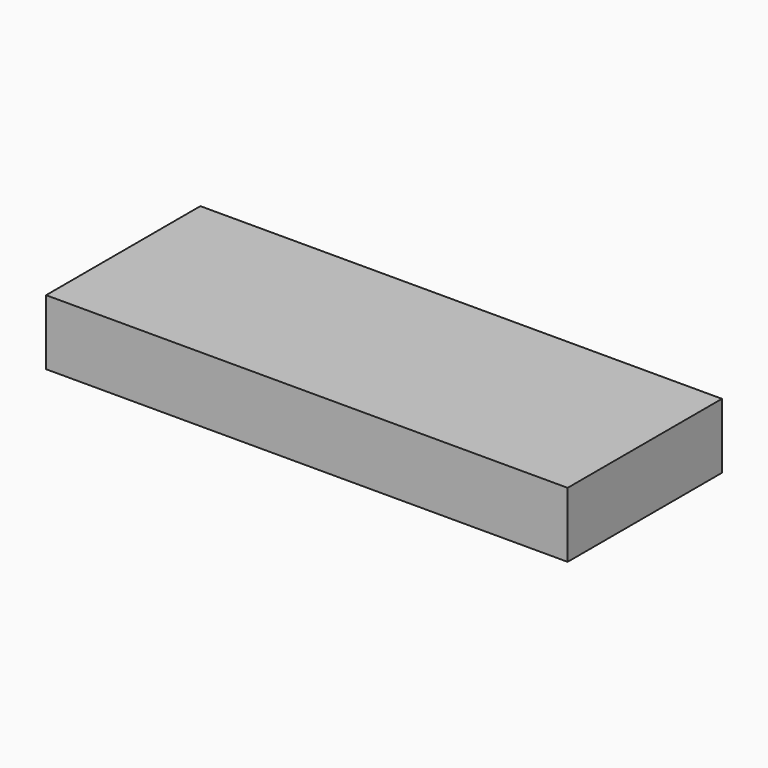
from build123d import *

# Parameters (mm, degrees)
F0_W      = 122.5
F0_H      = 57
F1_DEPTH  = 7
F2_R      = 5
F4_W      = 7.9906114999
F4_H      = 3.491573553
F6_DEPTH  = 0.75
F3_R      = 2.8696252626
F3_R_2    = 3.0222724843
F3_W      = 6.7058205605
F3_H      = 3.0176183209
F7_DEPTH  = 0.75
F5_R      = 4.4116461286
F8_DEPTH  = 0.5
F10_W     = 10.931
F10_H     = 2.55831494
F11_DEPTH = 1
F12_R     = 2.4748812048
F13_DEPTH = 7
F14_W     = 9.2436559498
F14_H     = 3.1246161088
F15_DEPTH = 25


# Not quite as in the source:
# - a fillet or chamfer that OpenCascade refuses, or shapes differently, is made with other operations: its cross-section is extruded or revolved along the edge and cut away or added


with BuildPart() as f1:
    # F0 (on Top) → F1 (new body)
    with BuildSketch(Plane.XY):
        Rectangle(F0_W, F0_H)
    extrude(amount=F1_DEPTH)

    # F2
    f2_edges = [f1.edges().sort_by_distance(p)[0] for p in [
        (61.25, -28.5, 3.5),
        (61.25, 28.5, 3.5),
        (-61.25, -28.5, 3.5),
        (-61.25, 28.5, 3.5),
    ]]
    fillet(f2_edges, radius=F2_R)

    # F4 (on face) → F6 (join)
    with BuildSketch(Plane(origin=(-61.25, 0, 0), x_dir=(0, -1, 0), z_dir=(-1, 0, 0))):
        with Locations((-17.3388376055, 3.4486234912)):
            Rectangle(F4_W, F4_H)
    extrude(amount=F6_DEPTH)

    # F3 (on face) → F7 (join)
    with BuildSketch(Plane.XZ.offset(28.5)):
        with Locations((-42.9149009287, 3.2392428257)):
            Circle(F3_R)
        with Locations((-34.8679199815, 3.2392428257)):
            Circle(F3_R_2)
        with Locations((-51.1295311153, 3.2392428257)):
            Rectangle(F3_W, F3_H)
    extrude(amount=F7_DEPTH)

    # F5 (on face) → F8 (cut)
    with BuildSketch(Plane.XY.offset(7)):
        with Locations((54.2597770691, -0.2932948992)):
            Circle(F5_R)
    extrude(amount=-F8_DEPTH, mode=Mode.SUBTRACT)

    # F9: fillet of radius 1 on 1 edges, made by hand


with BuildPart() as f9_tool2:
    # F9_s3 → F9_t4 (revolve)
    with BuildSketch(Plane.XZ.offset(0.2932948992)):
        with BuildLine():
            ThreePointArc((58.6714231977, 7.5), (58.3785299789, 6.7928932188), (57.6714231977, 6.5))
            Line((57.6714231977, 6.5), (58.6714231977, 6.5))
            Line((58.6714231977, 6.5), (58.6714231977, 7.5))
        make_face()
    revolve(axis=Axis((54.2597770691, -0.2932948992, 6.5), (0, 0, 1)))

    split(bisect_by=Plane.XY.offset(7), keep=Keep.BOTTOM)


with BuildPart() as f1_1:
    add(f1.part)

    # F9_t1: union F9_tool2
    add(f9_tool2.part)

    # F10 (on face) → F11 (join)
    with BuildSketch(Plane.YZ.offset(61.25)):
        with Locations((-0.3508040114, 3.4726482118)):
            Rectangle(F10_W, F10_H)
    extrude(amount=-F11_DEPTH)

    # F12 (on face) → F13 (cut)
    with BuildSketch(Plane.YZ.offset(61.25)):
        with Locations((16.8605856597, 3.6920385901)):
            Circle(F12_R)
    extrude(amount=-F13_DEPTH, mode=Mode.SUBTRACT)

    # F14 (on face) → F15 (intersect)
    with BuildSketch(Plane.YZ.offset(61.25)):
        with Locations((0, 3.6012954079)):
            Rectangle(F14_W, F14_H)
    extrude(amount=-F15_DEPTH, mode=Mode.INTERSECT)


solid = f1_1.part
